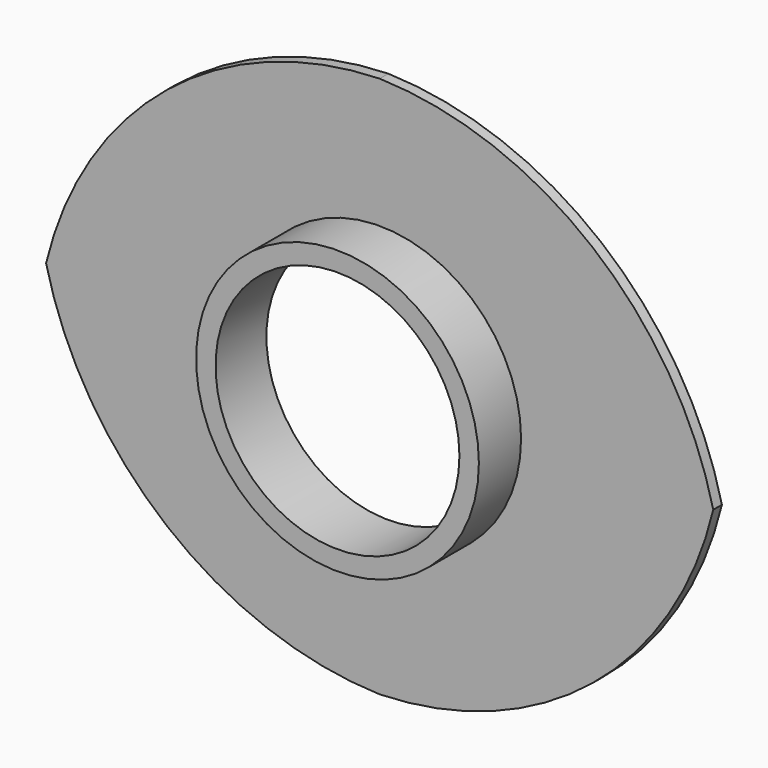
from build123d import *

# Parameters (mm, degrees)
F0_R        = 31.3722800925
F1_DEPTH    = 2.4
F0_R_2      = 27.0541255518
F2_DEPTH    = 14.1
F3_T1_DEPTH = 394.7097038856


# Not quite as in the source:
# - a fillet or chamfer that OpenCascade refuses, or shapes differently, is made with other operations: its cross-section is extruded or revolved along the edge and cut away or added


with BuildPart() as f1:
    # F0 (on Front) → F1 (new body)
    with BuildSketch(Plane.XZ):
        Polygon((76.1774070561, 60.170147568), (-76.1774070561, 60.170147568), (-76.1774070561, 34.1583490372), (-76.1774070561, -34.1583490372), (-76.1774070561, -60.170147568), (76.1774070561, -60.170147568), (76.1774070561, -34.1583490372), (76.1774070561, 34.1583490372), align=None)
        Circle(F0_R, mode=Mode.SUBTRACT)
    extrude(amount=F1_DEPTH)

    # F0 (on Front) → F2 (join)
    with BuildSketch(Plane.XZ):
        Circle(F0_R)
        Circle(F0_R_2, mode=Mode.SUBTRACT)
    extrude(amount=F2_DEPTH)

    # F3: fillet of radius 78.4619407771 on 4 edges, made by hand

    # F3_s2 → F3_t1 (cut)
    with BuildSketch(Plane.XZ.offset(-196.1548519428)):
        with BuildLine():
            ThreePointArc((2.284533721, 60.170147568), (-53.1964366675, 37.1891771794), (-76.1774070561, -18.2917932091))
            Line((-76.1774070561, -18.2917932091), (-76.1774070561, 60.170147568))
            Line((-76.1774070561, 60.170147568), (2.284533721, 60.170147568))
        make_face()
        with BuildLine():
            ThreePointArc((-2.284533721, 60.170147568), (53.1964366675, 37.1891771794), (76.1774070561, -18.2917932091))
            Line((76.1774070561, -18.2917932091), (76.1774070561, 60.170147568))
            Line((76.1774070561, 60.170147568), (-2.284533721, 60.170147568))
        make_face()
        with BuildLine():
            ThreePointArc((76.1774070561, 18.2917932091), (53.1964366675, -37.1891771794), (-2.284533721, -60.170147568))
            Line((-2.284533721, -60.170147568), (76.1774070561, -60.170147568))
            Line((76.1774070561, -60.170147568), (76.1774070561, 18.2917932091))
        make_face()
        with BuildLine():
            ThreePointArc((-76.1774070561, 18.2917932091), (-53.1964366675, -37.1891771794), (2.284533721, -60.170147568))
            Line((2.284533721, -60.170147568), (-76.1774070561, -60.170147568))
            Line((-76.1774070561, -60.170147568), (-76.1774070561, 18.2917932091))
        make_face()
    extrude(amount=F3_T1_DEPTH, mode=Mode.SUBTRACT)


solid = f1.part
